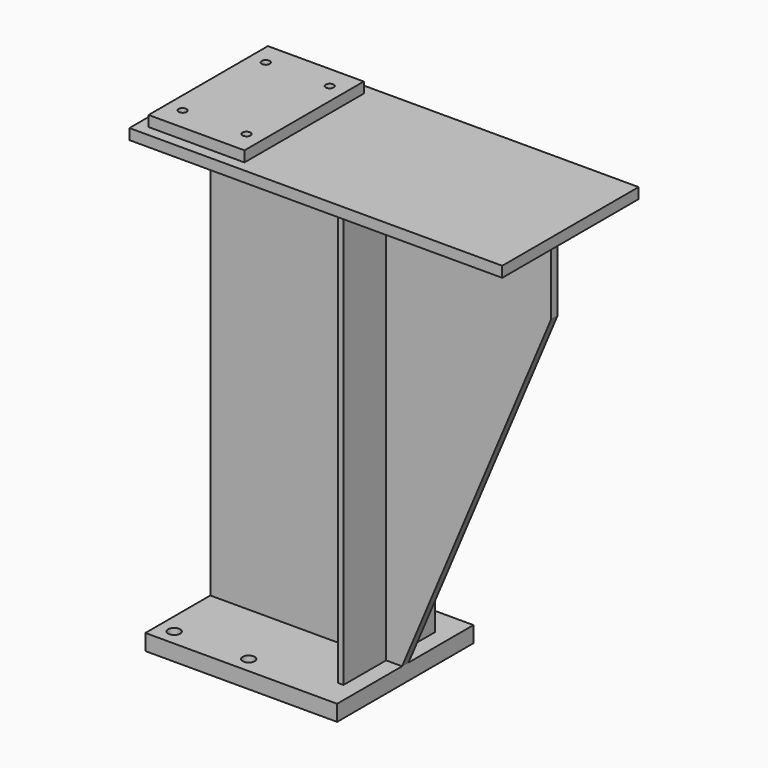
from build123d import *

# Parameters (mm, degrees)
F0_W      = 444.5
F0_H      = 203.2
F1_DEPTH  = 12.7
F2_W      = 114.3
F2_H      = 177.8
F3_DEPTH  = 12.7
F5_D      = 9.525
F6_W      = 203.2
F6_H      = 9.652
F6_W_2    = 6.35
F6_H_2    = 63.5
F6_W_3    = 196.85
F7_DEPTH  = 511.048
F9_DEPTH  = 106.427
F10_W     = 228.6
F10_H     = 203.2
F11_DEPTH = 19.05
F13_D     = 14.2875
F13_DEPTH = 31.75
F13_TIP   = 4.2923980472


# Not quite as in the source:
# - a length typed as a fraction of an inch, garbled in the dataset ("3 / 203.2 mm" for 3/8 in), is restored


with BuildPart() as f1:
    # F0 (on Top) → F1 (new body)
    with BuildSketch(Plane.XY):
        Rectangle(F0_W, F0_H)
    extrude(amount=F1_DEPTH)

    # F2 (on face) → F3 (join)
    with BuildSketch(Plane.XY.offset(12.7)):
        with Locations((-152.4, 0)):
            Rectangle(F2_W, F2_H)
    extrude(amount=F3_DEPTH)

    # F5 (through all)
    with Locations(Plane.XY.offset(25.4)):
        with Locations((-190.5, 61.976), (-114.3, 61.976), (-114.3, -61.976), (-190.5, -61.976)):
            Hole(F5_D / 2)

    # F6 (on face) → F7 (join)
    with BuildSketch(Plane(origin=(0, 0, 0), x_dir=(1, 0, 0), z_dir=(0, 0, -1))):
        with Locations((-101.6, 0)):
            Rectangle(F6_W, F6_H)
        with Locations((3.175, 0)):
            Rectangle(F6_W_2, F6_H)
        with Locations((3.175, -36.576)):
            Rectangle(F6_W_2, F6_H_2)
        with Locations((104.775, 0)):
            Rectangle(F6_W_3, F6_H)
        with Locations((3.175, 36.576)):
            Rectangle(F6_W_2, F6_H_2)
    extrude(amount=F7_DEPTH)

    # F8 (on face) → F9 (cut, through all)
    with BuildSketch(Plane.XZ.offset(4.826)):
        Polygon((203.2, -88.9), (25.4, -511.048), (203.2, -511.048), align=None)
    extrude(amount=-F9_DEPTH, mode=Mode.SUBTRACT)

    # F10 (on face) → F11 (join)
    with BuildSketch(Plane(origin=(0, 0, -511.048), x_dir=(1, 0, 0), z_dir=(0, 0, -1))):
        with Locations((-88.9, 0)):
            Rectangle(F10_W, F10_H)
    extrude(amount=F11_DEPTH)

    # F13
    with Locations(Plane(origin=(0, 0, -530.098), x_dir=(1, 0, 0), z_dir=(0, 0, -1))):
        with Locations((-184.15, 82.55), (-95.25, 82.55), (-95.25, -82.55), (-184.15, -82.55)):
            Hole(F13_D / 2, depth=F13_DEPTH)
            with Locations((0, 0, -(F13_DEPTH + F13_TIP / 2))):  # 118° drill point
                Cone(0, F13_D / 2, F13_TIP, mode=Mode.SUBTRACT)


solid = f1.part
